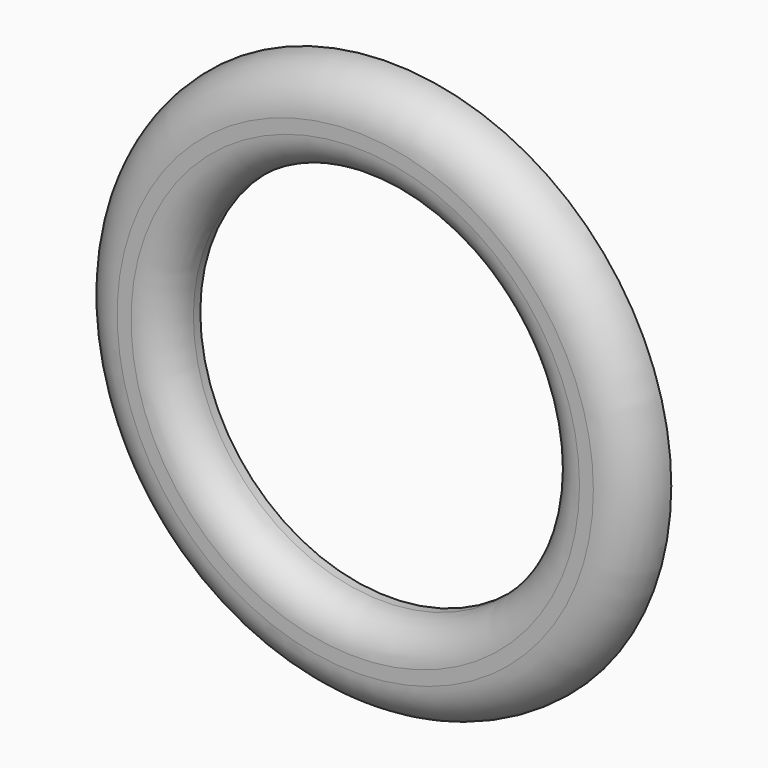
from build123d import *

# Parameters (mm, degrees)
F0_R     = 3.25
F0_R_2   = 2.19
F1_DEPTH = 0.5
F2_R     = 0.49999
F3_R     = 0.4


# Not quite as in the source:
# - a fillet or chamfer is up to 0.001 mm smaller than in the source, because OpenCascade refuses the exact size


with BuildPart() as f1:
    # F0 (on Front) → F1 (new body)
    with BuildSketch(Plane.XZ):
        Circle(F0_R)
        Circle(F0_R_2, mode=Mode.SUBTRACT)
    extrude(amount=F1_DEPTH)

    # F2 (radius 0.5 in the source; OpenCascade refuses exactly that, so slightly less here)
    f2_edges = [f1.edges().sort_by_distance(p)[0] for p in [
        (-3.25, -0.5, 0),
    ]]
    fillet(f2_edges, radius=F2_R)

    # F3
    f3_edges = [f1.edges().sort_by_distance(p)[0] for p in [
        (-2.19, -0.5, 0),
    ]]
    fillet(f3_edges, radius=F3_R)


solid = f1.part
